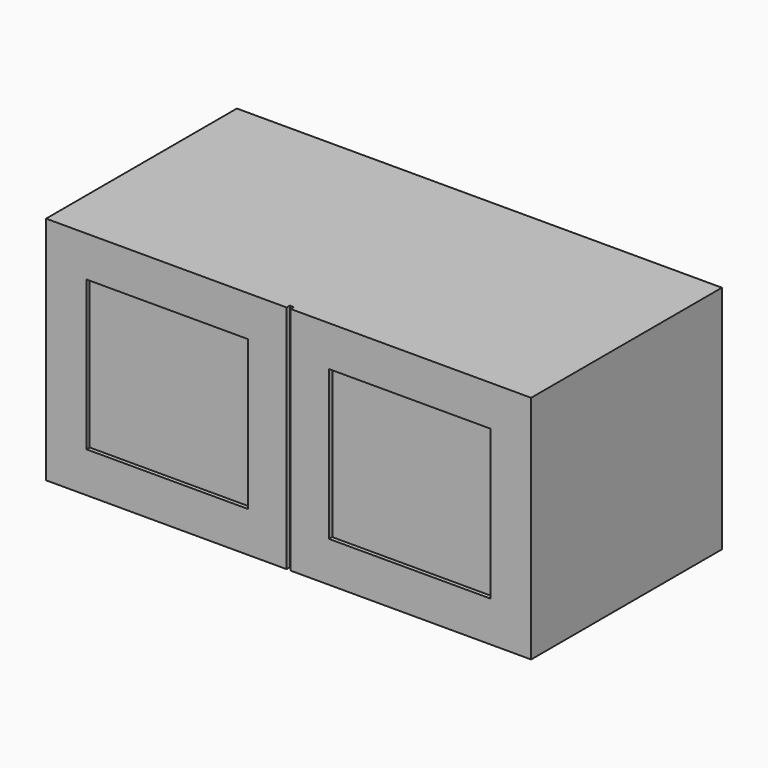
from build123d import *

# Parameters (mm, degrees)
F0_W     = 254
F0_H     = 234.95
F0_W_2   = 3.175
F0_H_2   = 361.95
F1_DEPTH = 374.65
F2_DEPTH = 6.35


# Not quite as in the source:
# - a feature names something its author has since deleted; it is built from what else it names


with BuildPart() as f1:
    # F0 (on Front) → F1 (new body)
    with BuildSketch(Plane.XZ):
        Polygon((-153.0927574873, 0), (224.7322425127, 0), (224.7322425127, 361.95), (177.1072425127, 361.95), (-153.0927574873, 361.95), align=None)
        with Locations((37.4072425127, 180.975)):
            Rectangle(F0_W, F0_H, mode=Mode.SUBTRACT)
        Polygon((231.0822425127, 361.95), (231.0822425127, 0), (608.9072425127, 0), (608.9072425127, 361.95), (278.7072425127, 361.95), align=None)
        with Locations((418.4072425127, 180.975)):
            Rectangle(F0_W, F0_H, mode=Mode.SUBTRACT)
        with Locations((37.4072425127, 180.975)):
            Rectangle(F0_W, F0_H)
        with Locations((418.4072425127, 180.975)):
            Rectangle(F0_W, F0_H)
        with Locations((226.3197425127, 180.975)):
            Rectangle(F0_W_2, F0_H_2)
        with Locations((229.4947425127, 180.975)):
            Rectangle(F0_W_2, F0_H_2)
    extrude(amount=-F1_DEPTH)

    # F0 (on Front) → F2 (cut)
    with BuildSketch(Plane.XZ):
        with Locations((226.3197425127, 180.975)):
            Rectangle(F0_W_2, F0_H_2)
        with Locations((229.4947425127, 180.975)):
            Rectangle(F0_W_2, F0_H_2)
        with Locations((37.4072425127, 180.975)):
            Rectangle(F0_W, F0_H)
        with Locations((418.4072425127, 180.975)):
            Rectangle(F0_W, F0_H)
    extrude(amount=-F2_DEPTH, mode=Mode.SUBTRACT)


solid = f1.part
